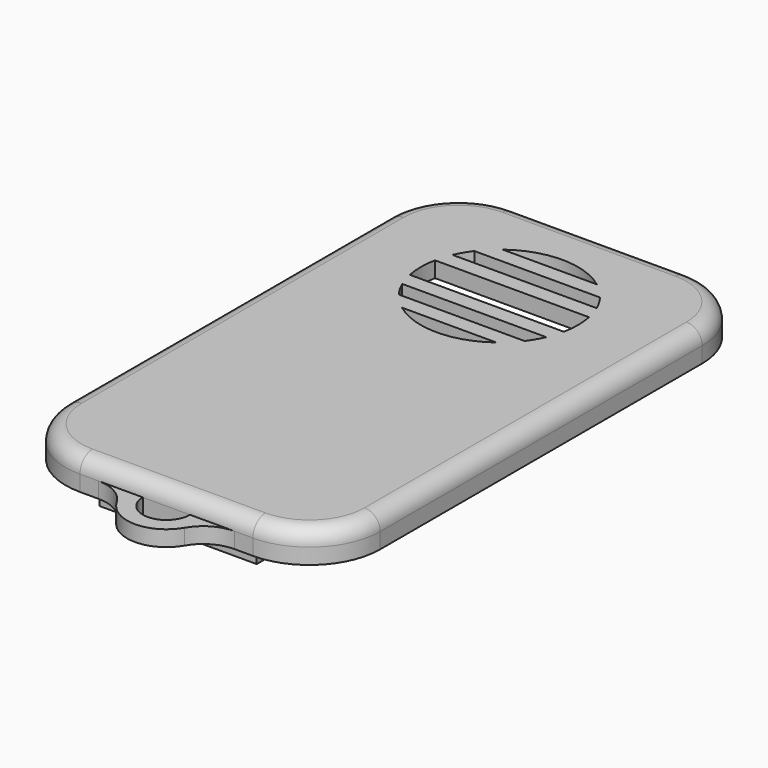
from build123d import *

# Parameters (mm, degrees)
F0_W      = 40
F0_H      = 69.2
F0_W_2    = 36
F0_H_2    = 65.2
F1_DEPTH  = 2
F2_W      = 20
F2_H      = 2
F3_DEPTH  = 2
F4_W      = 40
F4_H      = 69.2
F5_DEPTH  = 2
F6_R      = 7.99999
F7_R      = 9
F8_R      = 2
F10_DEPTH = 2
F11_R     = 5


# Not quite as in the source:
# - a fillet or chamfer is up to 0.001 mm smaller than in the source, because OpenCascade refuses the exact size


with BuildPart() as f1:
    # F0 (on Top) → F1 (new body)
    with BuildSketch(Plane.XY):
        with Locations((0, 0.4)):
            Rectangle(F0_W, F0_H)
        with Locations((0, 0.4)):
            Rectangle(F0_W_2, F0_H_2, mode=Mode.SUBTRACT)
    extrude(amount=F1_DEPTH)

    # F2 (on Top) → F3 (join, symmetric)
    with BuildSketch(Plane.XY):
        with Locations((0, -31.35)):
            Rectangle(F2_W, F2_H)
        with Locations((0, 32.15)):
            Rectangle(F2_W, F2_H)
    extrude(amount=F3_DEPTH, both=True)

    # F4 (on face) → F5 (join)
    with BuildSketch(Plane.XY.offset(2)):
        with Locations((0, 0.4)):
            Rectangle(F4_W, F4_H)
        with BuildLine():
            ThreePointArc((6, 10.7552776188), (0, 8.7552776188), (-6, 10.7552776188))
            Line((-6, 10.7552776188), (6, 10.7552776188))
        make_face(mode=Mode.SUBTRACT)
        with BuildLine():
            ThreePointArc((-8, 12.7552776188), (-8.6406368723, 13.721452588), (-9.1651513899, 14.7552776188))
            Line((-9.1651513899, 14.7552776188), (9.1651513899, 14.7552776188))
            ThreePointArc((9.1651513899, 14.7552776188), (8.6406368723, 13.721452588), (8, 12.7552776188))
            Line((8, 12.7552776188), (-8, 12.7552776188))
        make_face(mode=Mode.SUBTRACT)
        with BuildLine():
            Line((9.7979589711, 16.7552776188), (-9.7979589711, 16.7552776188))
            ThreePointArc((-9.7979589711, 16.7552776188), (-10, 18.7552776188), (-9.7979589711, 20.7552776188))
            Line((-9.7979589711, 20.7552776188), (9.7979589711, 20.7552776188))
            ThreePointArc((9.7979589711, 20.7552776188), (10, 18.7552776188), (9.7979589711, 16.7552776188))
        make_face(mode=Mode.SUBTRACT)
        with BuildLine():
            Line((9.1651513899, 22.7552776188), (-9.1651513899, 22.7552776188))
            ThreePointArc((-9.1651513899, 22.7552776188), (-8.6406368723, 23.7891026495), (-8, 24.7552776188))
            Line((-8, 24.7552776188), (8, 24.7552776188))
            ThreePointArc((8, 24.7552776188), (8.6406368723, 23.7891026495), (9.1651513899, 22.7552776188))
        make_face(mode=Mode.SUBTRACT)
        with BuildLine():
            Line((6, 26.7552776188), (-6, 26.7552776188))
            ThreePointArc((-6, 26.7552776188), (0, 28.7552776188), (6, 26.7552776188))
        make_face(mode=Mode.SUBTRACT)
    extrude(amount=F5_DEPTH)

    # F6 (radius 8 in the source; OpenCascade refuses exactly that, so slightly less here)
    f6_edges = [f1.edges().sort_by_distance(p)[0] for p in [
        (18, 33, 1),
        (-18, 33, 1),
        (18, -32.2, 1),
        (-18, -32.2, 1),
    ]]
    fillet(f6_edges, radius=F6_R)

    # F7
    f7_edges = [f1.edges().sort_by_distance(p)[0] for p in [
        (-20, -34.2, 2),
        (-20, 35, 2),
        (20, 35, 2),
        (20, -34.2, 2),
    ]]
    fillet(f7_edges, radius=F7_R)

    # F8
    f8_edges = [f1.edges().sort_by_distance(p)[0] for p in [
        (20, 0.4, 4),
    ]]
    fillet(f8_edges, radius=F8_R)

    # F9 (on face) → F10 (join)
    with BuildSketch(Plane(origin=(0, 0, 0), x_dir=(1, 0, 0), z_dir=(0, 0, -1))):
        with BuildLine():
            Line((3, 34.2), (5, 34.2))
            ThreePointArc((5, 34.2), (0, 39.2), (-5, 34.2))
            Line((-5, 34.2), (-3, 34.2))
            ThreePointArc((-3, 34.2), (0, 37.2), (3, 34.2))
        make_face()
    extrude(amount=-F10_DEPTH)

    # F11
    f11_edges = [f1.edges().sort_by_distance(p)[0] for p in [
        (-5, -34.2, 1),
        (5, -34.2, 1),
    ]]
    fillet(f11_edges, radius=F11_R)


solid = f1.part
